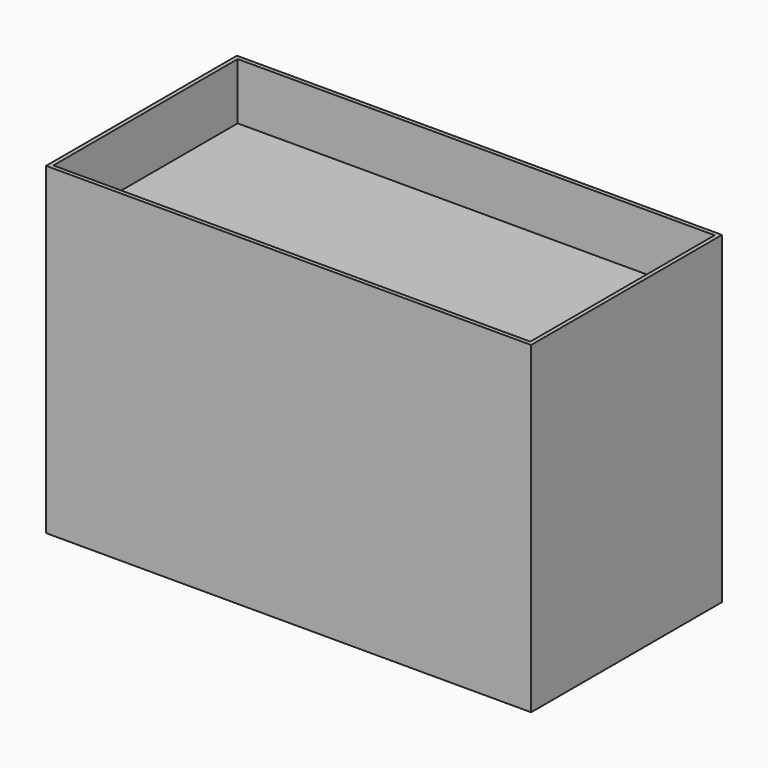
from build123d import *

# Parameters (mm, degrees)
F0_W     = 600
F0_H     = 295
F1_DEPTH = 400
F2_T     = -5
F3_W     = 590
F3_H     = 285
F4_DEPTH = 325


with BuildPart() as f1:
    # F0 (on Top) → F1 (new body)
    with BuildSketch(Plane.XY):
        Rectangle(F0_W, F0_H)
    extrude(amount=F1_DEPTH)

    # F2
    f2_openings = [f1.faces().sort_by_distance(p)[0] for p in [
        (0, 0, 400),
    ]]
    offset(amount=F2_T, openings=f2_openings)


with BuildPart() as f4:
    # F3 (on face) → F4 (new body)
    with BuildSketch(Plane.XY.offset(5)):
        Rectangle(F3_W, F3_H)
    extrude(amount=F4_DEPTH)


solid = Compound([f1.part, f4.part])
